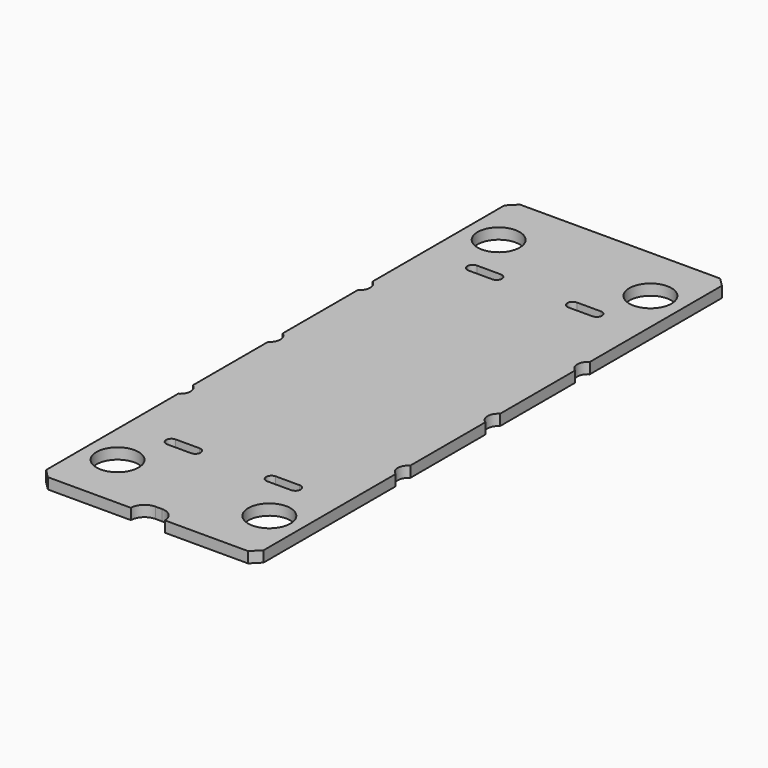
from build123d import *

# Parameters (mm, degrees)
F0_W     = 32
F0_H     = 86.86
F1_DEPTH = 1.6
F2_R     = 3.1
F2_R_2   = 1.585
F2_W     = 5
F2_H     = 2.4618506432
F3_DEPTH = 25
F4_SIZE  = 1.27
F5_R     = 1.99999


# Not quite as in the source:
# - a fillet or chamfer is up to 0.001 mm smaller than in the source, because OpenCascade refuses the exact size


with BuildPart() as f1:
    # F0 (on Top) → F1 (new body)
    with BuildSketch(Plane.XY):
        Rectangle(F0_W, F0_H)
    extrude(amount=F1_DEPTH)

    # F2 (on face) → F3 (cut)
    with BuildSketch(Plane.XY.offset(1.6)):
        with Locations((-11.17, 35.05)):
            Circle(F2_R)
        with Locations((11.17, 35.05)):
            Circle(F2_R)
        with Locations((-11.17, -35.05)):
            Circle(F2_R)
        with Locations((11.17, -35.05)):
            Circle(F2_R)
        with BuildLine():
            Line((9.115, 28.49), (5.605, 28.49))
            ThreePointArc((5.605, 28.49), (5.0499211768, 28.2600788232), (4.82, 27.705))
            ThreePointArc((4.82, 27.705), (5.0499211768, 27.1499211768), (5.605, 26.92))
            Line((5.605, 26.92), (9.115, 26.92))
            ThreePointArc((9.115, 26.92), (9.6700788232, 27.1499211768), (9.9, 27.705))
            ThreePointArc((9.9, 27.705), (9.6700788232, 28.2600788232), (9.115, 28.49))
        make_face()
        with BuildLine():
            Line((-5.605, 28.49), (-9.115, 28.49))
            ThreePointArc((-9.115, 28.49), (-9.6700788232, 28.2600788232), (-9.9, 27.705))
            ThreePointArc((-9.9, 27.705), (-9.6700788232, 27.1499211768), (-9.115, 26.92))
            Line((-9.115, 26.92), (-5.605, 26.92))
            ThreePointArc((-5.605, 26.92), (-5.0499211768, 27.1499211768), (-4.82, 27.705))
            ThreePointArc((-4.82, 27.705), (-5.0499211768, 28.2600788232), (-5.605, 28.49))
        make_face()
        with Locations((16.825, 16.51)):
            Circle(F2_R_2)
        with Locations((16.825, 0)):
            Circle(F2_R_2)
        with Locations((16.825, -16.51)):
            Circle(F2_R_2)
        with Locations((-16.825, 0)):
            Circle(F2_R_2)
        with Locations((-16.825, 16.51)):
            Circle(F2_R_2)
        with Locations((-16.825, -16.51)):
            Circle(F2_R_2)
        with BuildLine():
            Line((-5.605, -26.92), (-9.115, -26.92))
            ThreePointArc((-9.115, -26.92), (-9.6700788232, -27.1499211768), (-9.9, -27.705))
            ThreePointArc((-9.9, -27.705), (-9.6700788232, -28.2600788232), (-9.115, -28.49))
            Line((-9.115, -28.49), (-5.605, -28.49))
            ThreePointArc((-5.605, -28.49), (-5.0499211768, -28.2600788232), (-4.82, -27.705))
            ThreePointArc((-4.82, -27.705), (-5.0499211768, -27.1499211768), (-5.605, -26.92))
        make_face()
        with BuildLine():
            Line((9.115, -26.92), (5.605, -26.92))
            ThreePointArc((5.605, -26.92), (5.0499211768, -27.1499211768), (4.82, -27.705))
            ThreePointArc((4.82, -27.705), (5.0499211768, -28.2600788232), (5.605, -28.49))
            Line((5.605, -28.49), (9.115, -28.49))
            ThreePointArc((9.115, -28.49), (9.6700788232, -28.2600788232), (9.9, -27.705))
            ThreePointArc((9.9, -27.705), (9.6700788232, -27.1499211768), (9.115, -26.92))
        make_face()
        with Locations((0, -42.6609253216)):
            Rectangle(F2_W, F2_H)
    extrude(amount=-F3_DEPTH, mode=Mode.SUBTRACT)

    # F4
    f4_edges = [f1.edges().sort_by_distance(p)[0] for p in [
        (16, 43.43, 0.8),
        (-16, 43.43, 0.8),
        (16, -43.43, 0.8),
        (-16, -43.43, 0.8),
    ]]
    chamfer(f4_edges, length=F4_SIZE)

    # F5 (radius 2 in the source; OpenCascade refuses exactly that, so slightly less here)
    f5_edges = [f1.edges().sort_by_distance(p)[0] for p in [
        (-2.5, -41.43, 0.8),
        (2.5, -41.43, 0.8),
    ]]
    fillet(f5_edges, radius=F5_R)


solid = f1.part
